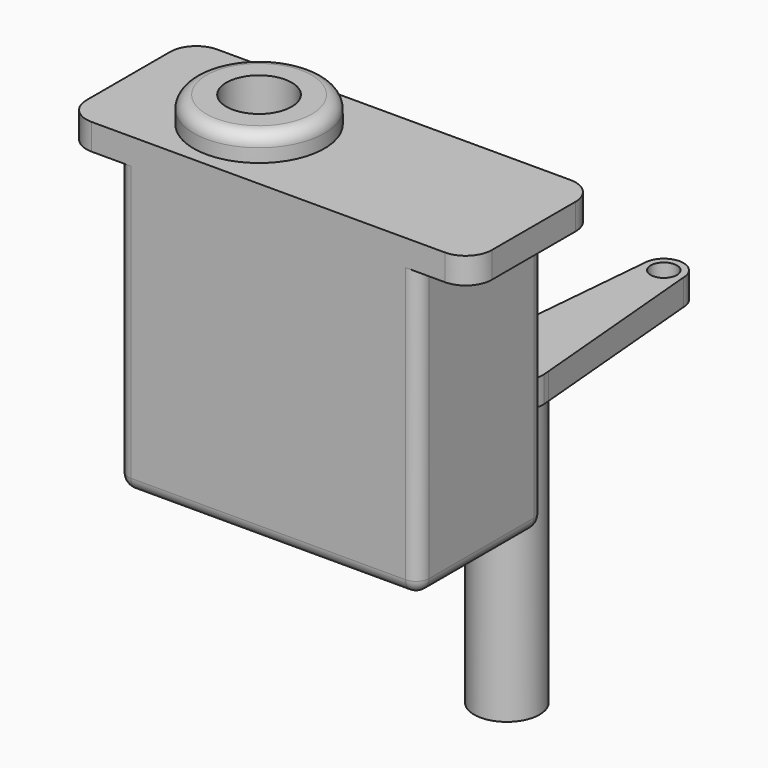
from build123d import *

# Parameters (mm, degrees)
F0_W      = 23
F0_H      = 22
F1_DEPTH  = 12
F2_R      = 1
F3_R      = 2
F5_DEPTH  = 2
F7_R      = 2.5
F8_DEPTH  = 20
F9_R      = 2.5
F10_DEPTH = 21
F12_DEPTH = 2


# Not quite as in the source:
# - a fillet or chamfer that OpenCascade refuses, or shapes differently, is made with other operations: its cross-section is extruded or revolved along the edge and cut away or added


with BuildPart() as f1:
    # F0 (on Front) → F1 (new body)
    with BuildSketch(Plane.XZ):
        Polygon((-53.2299494938, 49.2620729506), (-30.2299494938, 49.2620729506), (-26.2299494938, 49.2620729506), (-26.2299494938, 51.2620729506), (-57.2299494938, 51.2620729506), (-57.2299494938, 49.2620729506), align=None)
        with Locations((-41.7299494938, 38.2620729506)):
            Rectangle(F0_W, F0_H)
    extrude(amount=F1_DEPTH)

    # F2
    f2_edges = [f1.edges().sort_by_distance(p)[0] for p in [
        (-53.229949, -12, 38.262073),
        (-30.229949, -12, 38.262073),
        (-53.229949, 0, 38.262073),
        (-30.229949, 0, 38.262073),
        (-41.729949, -12, 27.262073),
        (-53.229949, -6, 27.262073),
        (-30.229949, -6, 27.262073),
        (-41.729949, 0, 27.262073),
    ]]
    fillet(f2_edges, radius=F2_R)

    # F3
    f3_edges = [f1.edges().sort_by_distance(p)[0] for p in [
        (-26.229949, -12, 50.262073),
        (-26.229949, 0, 50.262073),
        (-57.229949, -12, 50.262073),
        (-57.229949, 0, 50.262073),
    ]]
    fillet(f3_edges, radius=F3_R)

    # F4 (on face) → F5 (join)
    with BuildSketch(Plane.XY.offset(51.2620729506)):
        with BuildLine():
            ThreePointArc((-42.2299494938, -6), (-47.2299494938, -1), (-52.2299494938, -6))
            ThreePointArc((-52.2299494938, -6), (-47.2299494938, -11), (-42.2299494938, -6))
        make_face()
    extrude(amount=F5_DEPTH)

    # F6: fillet of radius 1 on 1 edges, made by hand

    # F6_s1 → F6_t2 (revolve, cut)
    with BuildSketch(Plane.XZ.offset(6)):
        with BuildLine():
            ThreePointArc((-42.2295494938, 52.2611072652), (-42.5228427126, 52.9691797318), (-43.2309151792, 53.2624729506))
            Line((-43.2309151792, 53.2624729506), (-43.2309151792, 53.3626095191))
            ThreePointArc((-43.2309151792, 53.3626095191), (-42.7304323365, 53.3622095191), (-42.2299494938, 53.3622095191))
            Line((-42.2299494938, 53.3622095191), (-42.1298129252, 53.2620729506))
            ThreePointArc((-42.1298129252, 53.2620729506), (-42.1298129252, 52.7615901079), (-42.1294129252, 52.2611072652))
            Line((-42.1294129252, 52.2611072652), (-42.2295494938, 52.2611072652))
        make_face()
    revolve(axis=Axis((-47.2299494938, -6, 53.2620729506), (0, 0, -1)), mode=Mode.SUBTRACT)

    # F7 (on face) → F8 (cut)
    with BuildSketch(Plane.XY.offset(53.2620729506)):
        with Locations((-47.2299494938, -6)):
            Circle(F7_R)
    extrude(amount=-F8_DEPTH, mode=Mode.SUBTRACT)


with BuildPart() as f10:
    # F9 (on Top) → F10 (new body)
    with BuildSketch(Plane.XY):
        with Locations((-50.499279052, 21.7643305659)):
            Circle(F9_R)
    extrude(amount=F10_DEPTH)

    # F11 (on face) → F12 (join)
    with BuildSketch(Plane.XY.offset(21)):
        with BuildLine():
            Line((-50.499279052, 35.2643305659), (-50.499279052, 24.5955677889))
            ThreePointArc((-50.499279052, 24.5955677889), (-48.6821090098, 23.9354586715), (-47.7122932643, 22.2629430725))
            Line((-47.7122932643, 22.2629430725), (-48.999279052, 36.7643305659))
            ThreePointArc((-48.999279052, 36.7643305659), (-49.4386188802, 35.7036703941), (-50.499279052, 35.2643305659))
        make_face()
        with BuildLine():
            ThreePointArc((-53.2862648398, 22.2629430725), (-52.3164490942, 23.9354586715), (-50.499279052, 24.5955677889))
            Line((-50.499279052, 24.5955677889), (-50.499279052, 35.2643305659))
            ThreePointArc((-50.499279052, 35.2643305659), (-51.5599392238, 35.7036703941), (-51.999279052, 36.7643305659))
            Line((-51.999279052, 36.7643305659), (-53.2862648398, 22.2629430725))
        make_face()
        with BuildLine():
            ThreePointArc((-47.7122932643, 22.2629430725), (-48.6821090098, 23.9354586715), (-50.499279052, 24.5955677889))
            ThreePointArc((-50.499279052, 24.5955677889), (-52.3164490942, 23.9354586715), (-53.2862648398, 22.2629430725))
            Line((-53.2862648398, 22.2629430725), (-53.330516275, 21.7643305659))
            ThreePointArc((-53.330516275, 21.7643305659), (-50.499279052, 18.9330933429), (-47.668041829, 21.7643305659))
            Line((-47.668041829, 21.7643305659), (-47.7122932643, 22.2629430725))
        make_face()
        with BuildLine():
            ThreePointArc((-47.999279052, 21.7643305659), (-52.267046005, 19.996563613), (-50.499279052, 24.2643305659))
            ThreePointArc((-50.499279052, 24.2643305659), (-48.7315120991, 23.5320975189), (-47.999279052, 21.7643305659))
        make_face(mode=Mode.SUBTRACT)
        with BuildLine():
            ThreePointArc((-47.999279052, 21.7643305659), (-48.7315120991, 23.5320975189), (-50.499279052, 24.2643305659))
            ThreePointArc((-50.499279052, 24.2643305659), (-52.267046005, 19.996563613), (-47.999279052, 21.7643305659))
        make_face()
        with BuildLine():
            ThreePointArc((-51.999279052, 36.7643305659), (-51.5599392238, 35.7036703941), (-50.499279052, 35.2643305659))
            ThreePointArc((-50.499279052, 35.2643305659), (-49.4386188802, 35.7036703941), (-48.999279052, 36.7643305659))
            ThreePointArc((-48.999279052, 36.7643305659), (-50.499279052, 38.2643305659), (-51.999279052, 36.7643305659))
        make_face()
        with BuildLine():
            ThreePointArc((-49.499279052, 36.7643305659), (-49.7921722708, 36.0572237847), (-50.499279052, 35.7643305659))
            ThreePointArc((-50.499279052, 35.7643305659), (-51.2063858332, 37.4714373471), (-49.499279052, 36.7643305659))
        make_face(mode=Mode.SUBTRACT)
    extrude(amount=F12_DEPTH)


solid = Compound([f1.part, f10.part])
